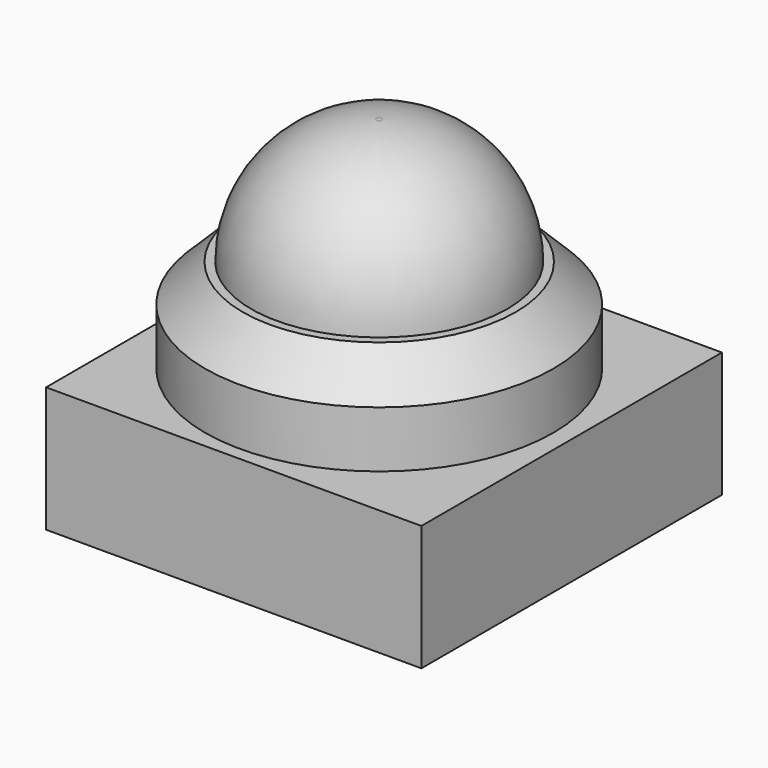
from build123d import *

# Parameters (mm, degrees)
F0_W     = 76.0409757495
F0_H     = 76.1161372066
F1_DEPTH = 25.4
F2_R     = 35.2777719823
F3_DEPTH = 19.05
F4_R     = 25.9547927972
F5_DEPTH = 25.4
F6_R     = 25.39999
F7_SIZE  = 7.62


# Not quite as in the source:
# - a fillet or chamfer is up to 0.001 mm smaller than in the source, because OpenCascade refuses the exact size


with BuildPart() as f1:
    # F0 (on Top) → F1 (new body)
    with BuildSketch(Plane.XY):
        with Locations((38.0204878747, -38.0580686033)):
            Rectangle(F0_W, F0_H)
    extrude(amount=F1_DEPTH)


with BuildPart() as f3:
    # F2 (on face) → F3 (new body)
    with BuildSketch(Plane.XY.offset(25.4)):
        with Locations((37.132114172, -38.1562672555)):
            Circle(F2_R)
    extrude(amount=F3_DEPTH)

    # F7
    f7_edges = [f3.edges().sort_by_distance(p)[0] for p in [
        (1.854342, -38.156267, 44.45),
    ]]
    chamfer(f7_edges, length=F7_SIZE)


with BuildPart() as f5:
    # F4 (on face) → F5 (new body)
    with BuildSketch(Plane.XY.offset(44.45)):
        with Locations((37.132114172, -38.1562672555)):
            Circle(F4_R)
    extrude(amount=F5_DEPTH)

    # F6 (radius 25.4 in the source; OpenCascade refuses exactly that, so slightly less here)
    f6_edges = [f5.edges().sort_by_distance(p)[0] for p in [
        (11.177321, -38.156267, 69.85),
    ]]
    fillet(f6_edges, radius=F6_R)


solid = Compound([f1.part, f3.part, f5.part])
